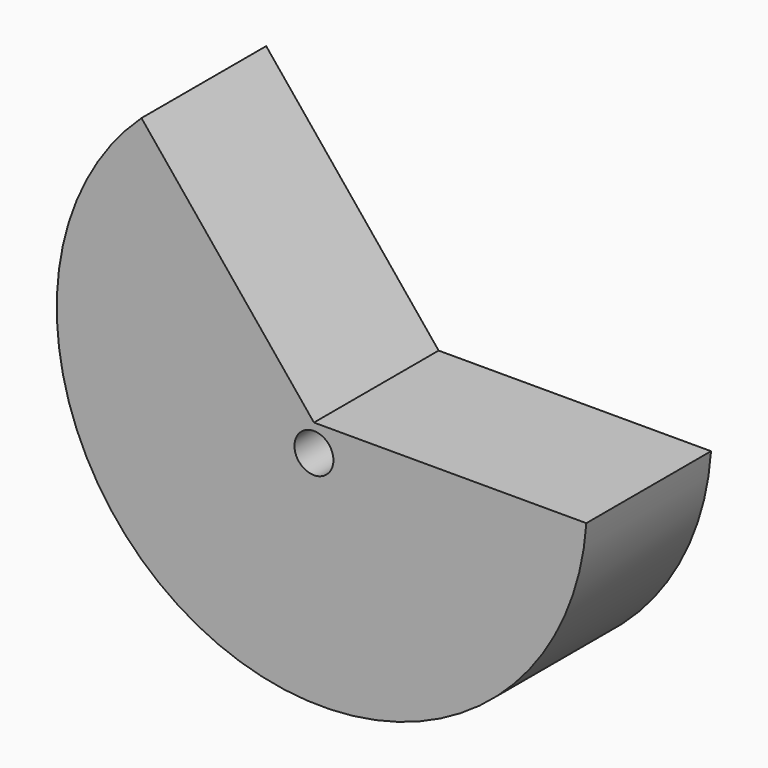
from build123d import *

# Parameters (mm, degrees)
F0_R     = 3.175
F1_DEPTH = 25.4


# Not quite as in the source:
# - a feature names something its author has since deleted; it is built from what else it names


with BuildPart() as f1:
    # F0 (on Front) → F1 (new body)
    with BuildSketch(Plane.XZ):
        with BuildLine():
            Line((44.3896651268, 4.3802629225), (0, 4.3802629225))
            Line((0, 4.3802629225), (-28.1046908349, 38.9245525002))
            ThreePointArc((-28.1046908349, 38.9245525002), (-17.2982990716, -31.7374125613), (44.3896651268, 4.3802629225))
        make_face()
        Circle(F0_R, mode=Mode.SUBTRACT)
    extrude(amount=F1_DEPTH)


solid = f1.part
